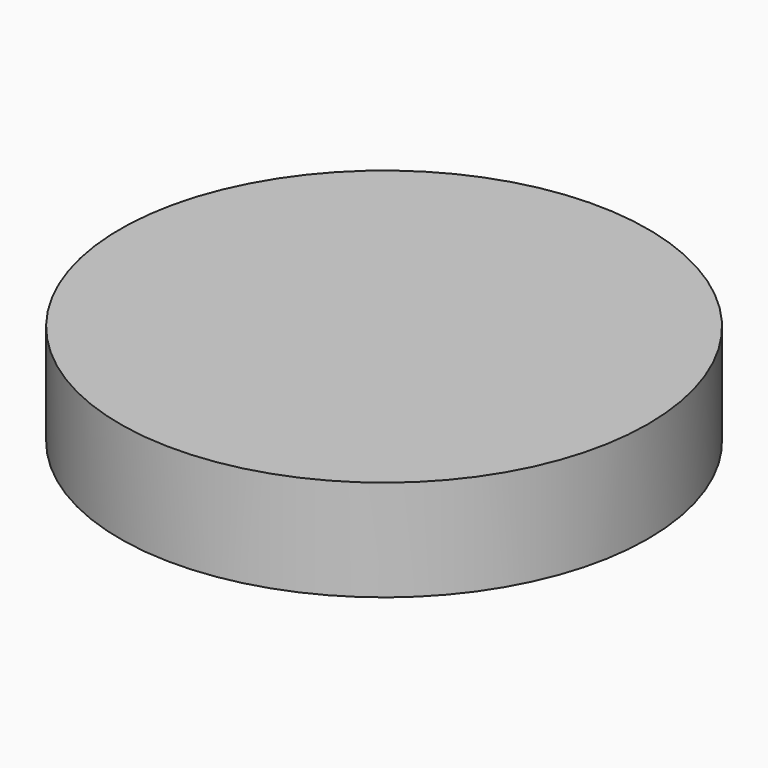
from build123d import *

# Parameters (mm, degrees)
F0_R     = 12.446
F2_DEPTH = 4.7625


# Not quite as in the source:
# - a length typed as a fraction of an inch, garbled in the dataset ("3 / 203.2 mm" for 3/8 in), is restored
# - the program builds the solid bodies; features that only make, move or delete a surface that nothing else refers to are left out


with BuildPart() as f2:
    # F0 (on Top) → F2 (new body)
    with BuildSketch(Plane.XY):
        with Locations((-40.744587779, 28.7767071277)):
            Circle(F0_R)
    extrude(amount=F2_DEPTH)


solid = f2.part
